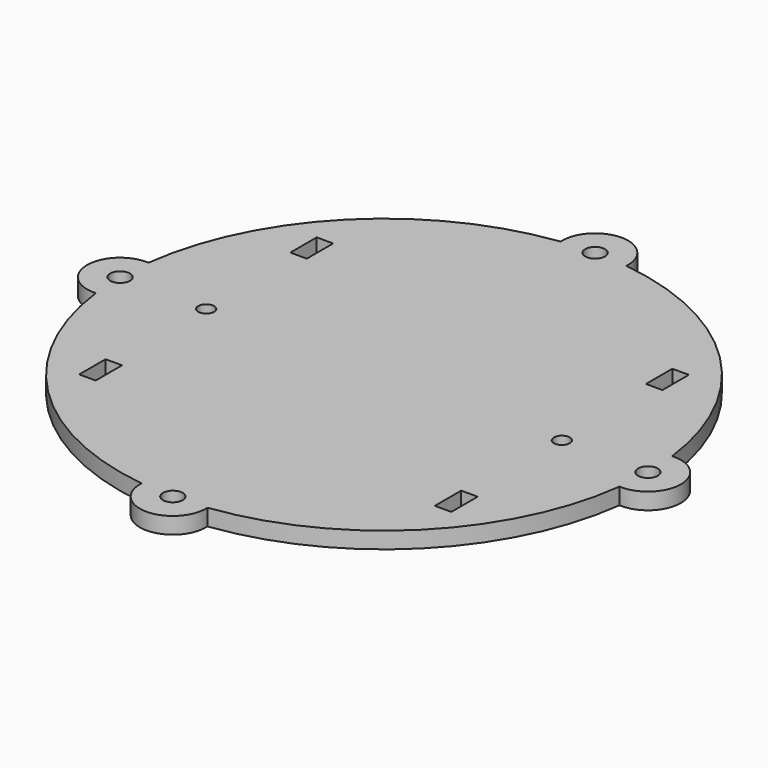
from build123d import *

# Parameters (mm, degrees)
F0_W     = 3.175
F0_H     = 6.35
F0_R     = 1.905
F0_R_2   = 1.524
F1_DEPTH = 3.175


# Not quite as in the source:
# - a length typed as a fraction of an inch, garbled in the dataset ("3 / 203.2 mm" for 3/8 in), is restored


with BuildPart() as f1:
    # F0 (on Top) → F1 (new body)
    with BuildSketch(Plane.XY):
        with BuildLine():
            ThreePointArc((-50.403125, 6.3375855209), (-57.15, 0), (-50.403125, -6.3375855209))
            ThreePointArc((-50.403125, -6.3375855209), (-35.9210244843, -35.9210244843), (-6.3375855209, -50.403125))
            ThreePointArc((-6.3375855209, -50.403125), (0, -57.15), (6.3375855209, -50.403125))
            ThreePointArc((6.3375855209, -50.403125), (35.9210244843, -35.9210244843), (50.403125, -6.3375855209))
            ThreePointArc((50.403125, -6.3375855209), (57.15, 0), (50.403125, 6.3375855209))
            ThreePointArc((50.403125, 6.3375855209), (35.9210244843, 35.9210244843), (6.3375855209, 50.403125))
            ThreePointArc((6.3375855209, 50.403125), (0, 57.15), (-6.3375855209, 50.403125))
            ThreePointArc((-6.3375855209, 50.403125), (-35.9210244843, 35.9210244843), (-50.403125, 6.3375855209))
        make_face()
        with Locations((-34.2304483056, -25.4)):
            Rectangle(F0_W, F0_H, mode=Mode.SUBTRACT)
        with Locations((0, -50.8)):
            Circle(F0_R, mode=Mode.SUBTRACT)
        with Locations((34.2304483056, -25.4)):
            Rectangle(F0_W, F0_H, mode=Mode.SUBTRACT)
        with Locations((-50.8, 0)):
            Circle(F0_R, mode=Mode.SUBTRACT)
        with Locations((-34.2304483056, 0)):
            Circle(F0_R_2, mode=Mode.SUBTRACT)
        with Locations((-34.2304483056, 25.4)):
            Rectangle(F0_W, F0_H, mode=Mode.SUBTRACT)
        with Locations((34.2304483056, 0)):
            Circle(F0_R_2, mode=Mode.SUBTRACT)
        with Locations((50.8, 0)):
            Circle(F0_R, mode=Mode.SUBTRACT)
        with Locations((34.2304483056, 25.4)):
            Rectangle(F0_W, F0_H, mode=Mode.SUBTRACT)
        with Locations((0, 50.8)):
            Circle(F0_R, mode=Mode.SUBTRACT)
    extrude(amount=F1_DEPTH)


solid = f1.part
